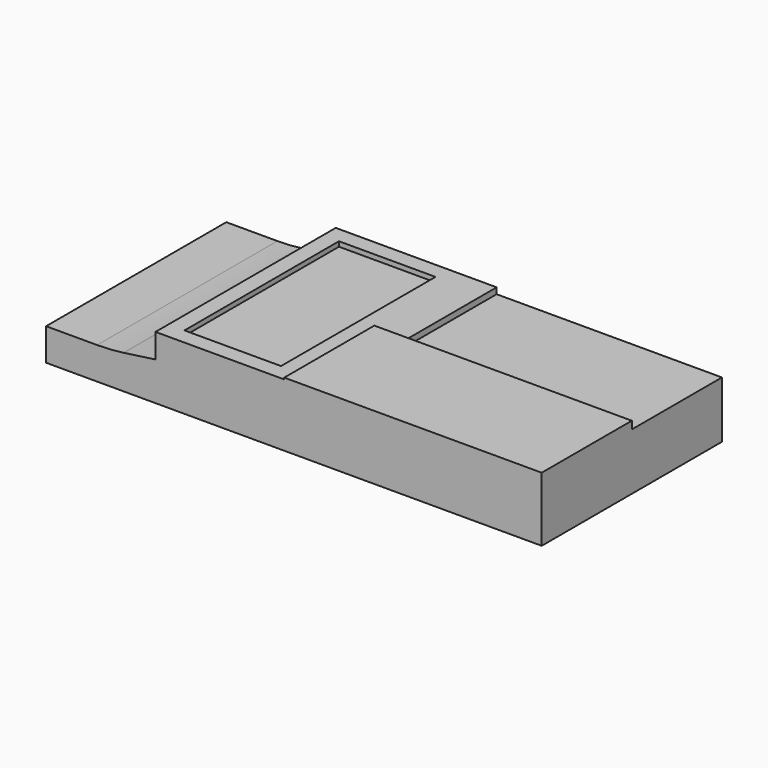
from build123d import *

# Parameters (mm, degrees)
F0_W          = 137.16
F0_H          = 177.8
F1_DEPTH      = 25.4
F3_DEPTH      = 177.801
F4_DEPTH      = 25.4
F5_DEPTH      = 203.2
F7_DEPTH      = 177.801
F8_W          = 88.9
F8_H          = 6.0689005345
F9_DEPTH      = 203.2010001
F10_T4_DEPTH  = 183.39269854
F10_T11_DEPTH = 88.9
F10_T16_DEPTH = 88.9
F11_DEPTH     = 50.8
F12_R         = 152.4
F13_W         = 101.6
F13_H         = 177.8
F14_DEPTH     = 50.8
F15_W         = 76.2
F15_H         = 152.4
F16_DEPTH     = 5.08
F17_DEPTH     = 25.4
F19_DEPTH     = 1.27
F20_DEPTH     = 25.4


# Not quite as in the source:
# - a fillet or chamfer that OpenCascade refuses, or shapes differently, is made with other operations: its cross-section is extruded or revolved along the edge and cut away or added


with BuildPart() as f1:
    # F0 (on Top) → F1 (new body)
    with BuildSketch(Plane.XY):
        Rectangle(F0_W, F0_H)
    extrude(amount=F1_DEPTH)

    # F2 (on face) → F3 (cut, through all)
    with BuildSketch(Plane.XZ.offset(88.9)):
        Polygon((-97.1020311117, 25.4), (-68.58, 0), (68.58, 25.4), (26.2377727777, 59.2203438282), align=None)
    extrude(amount=-F3_DEPTH, mode=Mode.SUBTRACT)

    # F4 (add): a face of the model
    f4_faces = [f1.faces().sort_by_distance(p)[0] for p in [
        (0, 0, 0),
    ]]
    extrude(f4_faces, amount=F4_DEPTH)

    # F5 (add): a face of the model
    f5_faces = [f1.faces().sort_by_distance(p)[0] for p in [
        (68.58, 0, 0),
    ]]
    extrude(f5_faces, amount=F5_DEPTH)

    # F6 (on face) → F7 (cut, through all)
    with BuildSketch(Plane(origin=(0, 88.9, 0), x_dir=(-1, 0, 0), z_dir=(0, 1, 0))):
        with BuildLine():
            add(Edge.make_bspline(
                [(68.58, 0), (45.7187770864, 3.1689187819), (-0.0085622279, 9.5074346586), (-45.7212234372, 16.0563109217), (-68.58, 19.3310994655)],
                knots=[0, 0, 0, 0, 0.4999464928, 1, 1, 1, 1], degree=3))
            Line((68.58, 0), (68.58, 17.6316630095))
            Line((68.58, 17.6316630095), (-68.58, 25.4))
            add(Edge.make_bspline(
                [(-68.58, 19.3310994655), (-68.58, 21.3540663103), (-68.58, 23.3770331552), (-68.58, 25.4)],
                knots=[0, 0, 0, 0, 6.0689005345, 6.0689005345, 6.0689005345, 6.0689005345], degree=3))
        make_face()
    extrude(amount=-F7_DEPTH, mode=Mode.SUBTRACT)

    # F8 (on face) → F9 (cut, through all)
    with BuildSketch(Plane(origin=(68.58, 0, 0), x_dir=(0, -1, 0), z_dir=(-1, 0, 0))):
        with Locations((-44.45, 22.3655497327)):
            Rectangle(F8_W, F8_H)
    extrude(amount=-F9_DEPTH, mode=Mode.SUBTRACT)

    # F10: fillet of radius 127 on 2 edges, made by hand


with BuildPart() as f10_tool2:
    # F10_s3 → F10_t4 (new body)
    with BuildSketch(Plane.XZ.offset(-94.49269854)):
        with BuildLine():
            ThreePointArc((31.1637123625, 13.9794051724), (50.3142381771, 18.2403654673), (68.58, 25.4))
            Line((68.58, 25.4), (69.6868281979, 23.1138391701))
            ThreePointArc((69.6868281979, 23.1138391701), (71.12, 22.3655497327), (71.12, 19.3310994655))
            Line((71.12, 19.3310994655), (68.9402072085, 16.8167703767))
            ThreePointArc((68.9402072085, 16.8167703767), (50.2320909574, 14.1376913402), (31.5222148076, 11.4648324459))
            Line((31.5222148076, 11.4648324459), (31.1637123625, 13.9794051724))
        make_face()
    extrude(amount=F10_T4_DEPTH)

    split(bisect_by=Plane.XZ.offset(-88.9), keep=Keep.TOP)

    split(bisect_by=Plane.XY.offset(19.3310994655), keep=Keep.BOTTOM)

    split(bisect_by=Plane.XZ, keep=Keep.BOTTOM)


with BuildPart() as f1_1:
    add(f1.part)

    # F10_t1: union F10_tool2
    add(f10_tool2.part)


with BuildPart() as f10_tool9:
    # F10_s10 → F10_t11 (new body)
    with BuildSketch(Plane.XZ):
        with BuildLine():
            ThreePointArc((31.1637123625, 13.9794051724), (50.3142381771, 18.2403654673), (68.58, 25.4))
            Line((68.58, 25.4), (69.6868281979, 23.1138391701))
            ThreePointArc((69.6868281979, 23.1138391701), (71.12, 22.3655497327), (71.12, 19.3310994655))
            Line((71.12, 19.3310994655), (68.9402072085, 16.8167703767))
            ThreePointArc((68.9402072085, 16.8167703767), (50.2320909574, 14.1376913402), (31.5222148076, 11.4648324459))
            Line((31.5222148076, 11.4648324459), (31.1637123625, 13.9794051724))
        make_face()
    extrude(amount=F10_T11_DEPTH)

    split(bisect_by=Plane.XY.offset(19.3310994655), keep=Keep.BOTTOM)


with BuildPart() as f1_2:
    add(f1_1.part)

    # F10_t8: union F10_tool9
    add(f10_tool9.part)


with BuildPart() as f10_tool14:
    # F10_s15 → F10_t16 (new body)
    with BuildSketch(Plane.XZ):
        with BuildLine():
            ThreePointArc((31.1637123625, 13.9794051724), (50.3142381771, 18.2403654673), (68.58, 25.4))
            Line((68.58, 25.4), (69.6868281979, 23.1138391701))
            ThreePointArc((69.6868281979, 23.1138391701), (71.12, 22.3655497327), (71.12, 19.3310994655))
            Line((71.12, 19.3310994655), (68.9402072085, 16.8167703767))
            ThreePointArc((68.9402072085, 16.8167703767), (50.2320909574, 14.1376913402), (31.5222148076, 11.4648324459))
            Line((31.5222148076, 11.4648324459), (31.1637123625, 13.9794051724))
        make_face()
    extrude(amount=F10_T16_DEPTH)

    split(bisect_by=Plane.XY.offset(19.3310994655), keep=Keep.TOP)


with BuildPart() as f1_3:
    add(f1_2.part)

    # F10_t13: union F10_tool14
    add(f10_tool14.part)

    # F11 (add): a face of the model
    f11_faces = [f1_3.faces().sort_by_distance(p)[0] for p in [
        (-68.58, 0, -12.7),
    ]]
    extrude(f11_faces, amount=F11_DEPTH)

    # F12
    f12_edges = [f1_3.edges().sort_by_distance(p)[0] for p in [
        (-68.58, 0, 0),
    ]]
    fillet(f12_edges, radius=F12_R)

    # F13 (on face) → F14 (join)
    with BuildSketch(Plane.XY.offset(25.4)):
        with Locations((17.78, 0)):
            Rectangle(F13_W, F13_H)
    extrude(amount=-F14_DEPTH)

    # F15 (on face) → F16 (cut)
    with BuildSketch(Plane.XY.offset(25.4)):
        with Locations((17.78, 0)):
            Rectangle(F15_W, F15_H)
    extrude(amount=-F16_DEPTH, mode=Mode.SUBTRACT)

    # F17 (add): a face of the model
    f17_faces = [f1_3.faces().sort_by_distance(p)[0] for p in [
        (68.58, 44.45, 22.3655497327),
    ]]
    extrude(f17_faces, amount=F17_DEPTH)

    # F18 (on face) → F19 (cut)
    with BuildSketch(Plane.XY.offset(25.4)):
        Polygon((93.98, -88.9), (93.98, 0), (93.98, 88.9), (-33.02, 88.9), (-33.02, -88.9), align=None)
    extrude(amount=-F19_DEPTH, mode=Mode.SUBTRACT)

    # F20 (add): a face of the model
    f20_faces = [f1_3.faces().sort_by_distance(p)[0] for p in [
        (93.98, -44.45, 24.765),
    ]]
    extrude(f20_faces, amount=F20_DEPTH)


solid = f1_3.part
